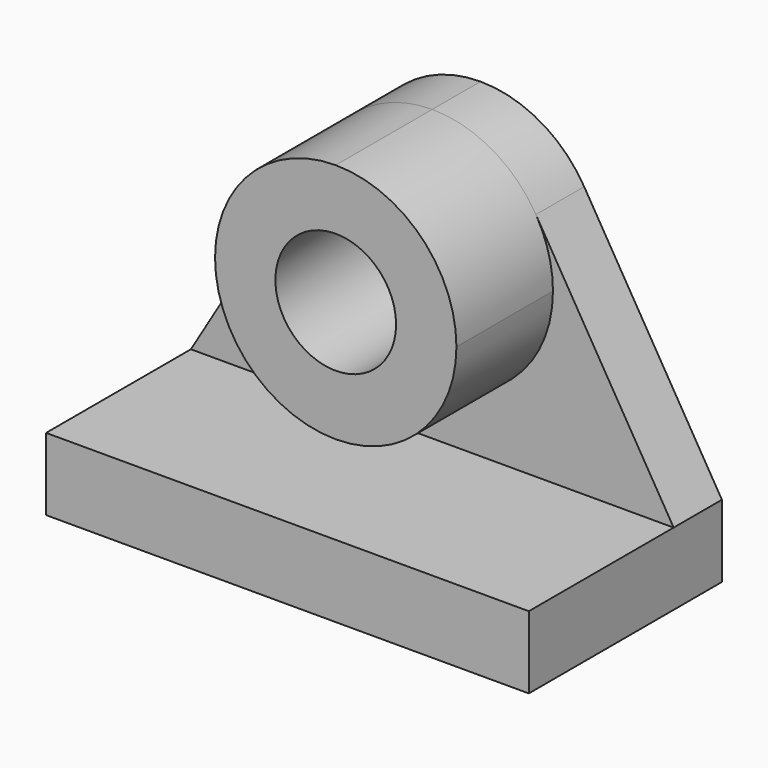
from build123d import *
from build123d import SkipClean  # not in build123d's __all__

# Parameters (mm, degrees)
F0_W      = 80
F0_H      = 40
F1_DEPTH  = 12
F2_W      = 80
F2_H      = 10
F3_DEPTH  = 48
F6_DEPTH  = 30
F7_R      = 10
F8_DEPTH  = 282
F10_DEPTH = 25


# Not quite as in the source:
# - a feature names something its author has since deleted; it is built from what else it names


with BuildPart() as f1:
    # F0 (on Top) → F1 (new body)
    with BuildSketch(Plane.XY):
        with Locations((15.4384085536, -20.999699384)):
            Rectangle(F0_W, F0_H)
    extrude(amount=F1_DEPTH)

    # F2 (on face) → F3 (join)
    with BuildSketch(Plane.XY.offset(12)):
        with Locations((15.4384085536, -5.999699384)):
            Rectangle(F2_W, F2_H)
    extrude(amount=F3_DEPTH)

    # F5 (on face) → F6 (join)
    with BuildSketch(Plane(origin=(0, -0.999699384, 0), x_dir=(-1, 0, 0), z_dir=(0, 1, 0))):
        with BuildLine():
            ThreePointArc((4.5615914464, 40), (-1.2962728753, 54.1421355692), (-15.4384083992, 60))
            ThreePointArc((-15.4384083992, 60), (-29.5805441228, 54.1421356783), (-35.4384085536, 40))
            Line((-35.4384085536, 40), (-25.4384085536, 40))
            ThreePointArc((-25.4384085536, 40), (-15.4384085536, 50), (-5.4384085536, 40))
            Line((-5.4384085536, 40), (4.5615914464, 40))
        make_face()
        with BuildLine():
            Line((-25.4384085536, 40), (-5.4384085536, 40))
            ThreePointArc((-5.4384085536, 40), (-15.4384085536, 50), (-25.4384085536, 40))
        make_face()
        with BuildLine():
            ThreePointArc((-25.4384085536, 40), (-15.4384085536, 30), (-5.4384085536, 40))
            Line((-5.4384085536, 40), (-25.4384085536, 40))
        make_face()
        with BuildLine():
            ThreePointArc((-35.4384085536, 40), (-15.4384085536, 20), (4.5615914464, 40))
            Line((4.5615914464, 40), (-5.4384085536, 40))
            ThreePointArc((-5.4384085536, 40), (-15.4384085536, 30), (-25.4384085536, 40))
            Line((-25.4384085536, 40), (-35.4384085536, 40))
        make_face()
    extrude(amount=-F6_DEPTH)

    # F7 (on face) → F8 (cut)
    with BuildSketch(Plane.XZ.offset(30.999699384)):
        with Locations((15.4384085536, 40)):
            Circle(F7_R)
    extrude(amount=-F8_DEPTH, mode=Mode.SUBTRACT)

    # F9 (on face) → F10 (cut)
    with BuildSketch(Plane.XZ.offset(10.999699384)):
        Polygon((55.4384085536, 60), (26.7936958102, 60), (32.6127306701, 50.2490321416), (55.4384085536, 12), align=None)
        with BuildLine():
            Line((32.6127306701, 50.2490321416), (26.7936958102, 60))
            Line((26.7936958102, 60), (15.4384085536, 60))
            ThreePointArc((15.4384085536, 60), (25.3131074647, 57.392248889), (32.6127306701, 50.2490321416))
        make_face()
        with BuildLine():
            ThreePointArc((-1.7359137949, 50.2490317528), (5.5637094457, 57.3922487772), (15.4384085536, 60))
            Line((15.4384085536, 60), (4.083121297, 60))
            Line((4.083121297, 60), (-1.7359137949, 50.2490317528))
        make_face()
        Polygon((-1.7359137949, 50.2490317528), (4.083121297, 60), (-24.5615914464, 60), (-24.5615914464, 12), align=None)
    with SkipClean():  # cleaning this boolean's faces spoils the solid; the shape is the same uncleaned
        extrude(amount=-F10_DEPTH, mode=Mode.SUBTRACT)


solid = f1.part
